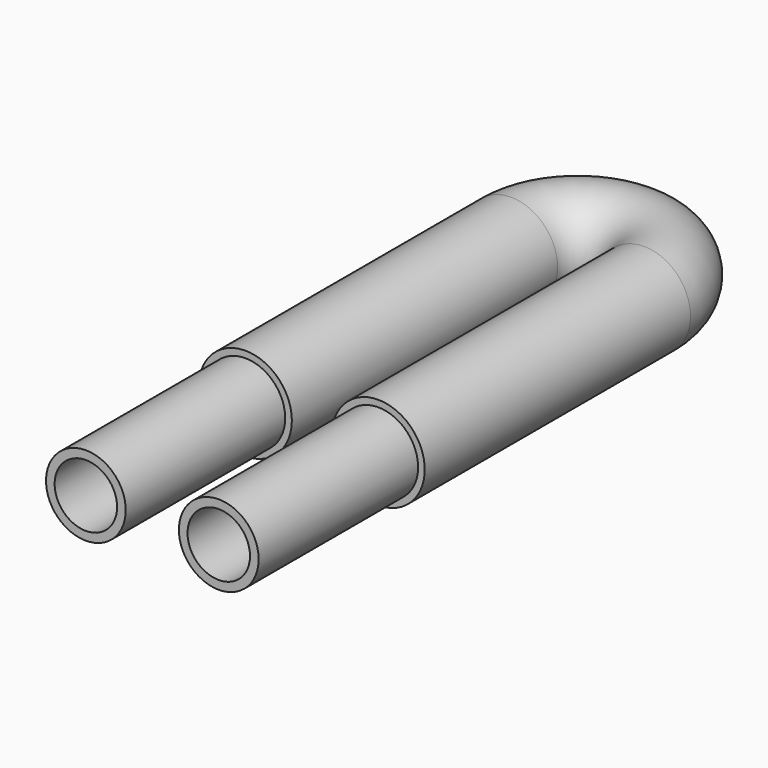
from build123d import *
from build123d import SkipClean  # not in build123d's __all__

# Parameters (mm, degrees)
F0_R     = 8.89
F0_R_2   = 5.969
F3_R     = 7.62
F3_R_2   = 5.969
F4_R     = 7.62
F4_R_2   = 5.969
F5_DEPTH = 38.1


with BuildPart() as f2:
    # F2: sweep along a path in F1
    with BuildLine(Plane.XY) as f2_path:
        Line((0, 0), (0, 63.5))
        ThreePointArc((0, 63.5), (12.7, 76.2), (25.4, 63.5))
        Line((25.4, 63.5), (25.4, 0))
    # F0 (on Front) → F2 (sweep)
    with BuildSketch(Plane.XZ):
        Circle(F0_R)
        Circle(F0_R_2, mode=Mode.SUBTRACT)
    sweep(path=f2_path.line)

    # F3 (on face) + F4 (on face) → F5 (join)
    with BuildSketch(Plane.XZ):
        Circle(F3_R)
        Circle(F3_R_2, mode=Mode.SUBTRACT)
    with BuildSketch(Plane.XZ):
        with Locations((25.4, 0)):
            Circle(F4_R)
        with Locations((25.4, 0)):
            Circle(F4_R_2, mode=Mode.SUBTRACT)
    with SkipClean():  # cleaning this boolean's faces spoils the solid; the shape is the same uncleaned
        extrude(amount=F5_DEPTH)


solid = f2.part
